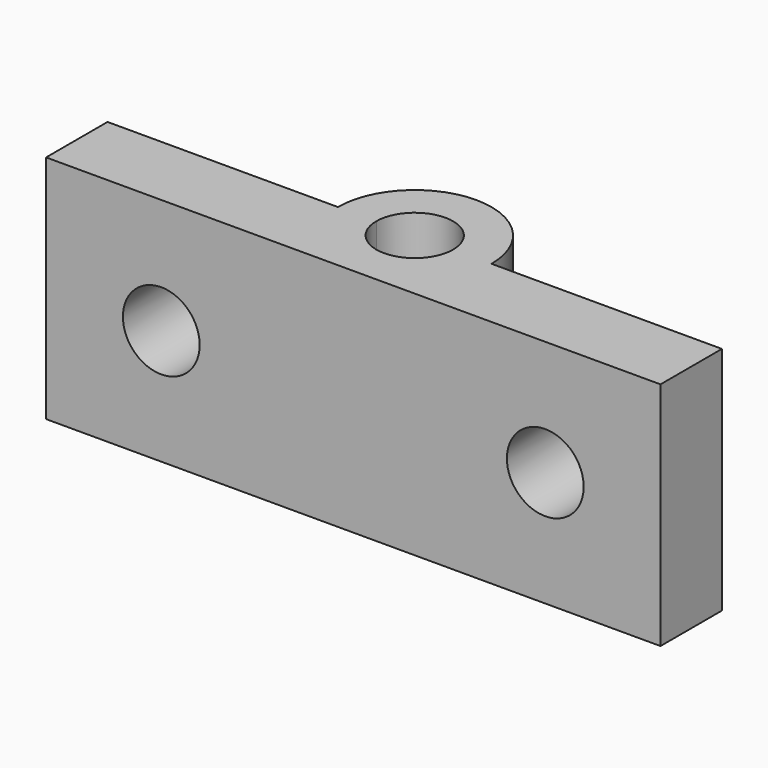
from build123d import *

# Parameters (mm, degrees)
F1_DEPTH = 9.525
F3_D     = 3.175
F5_D     = 3.175


# Not quite as in the source:
# - ends of sketch curves that miss each other by under 0.0002 mm in the source are joined
# - a length typed as a fraction of an inch, garbled in the dataset ("3 / 203.2 mm" for 3/8 in), is restored


with BuildPart() as f1:
    # F0 (on Top) → F1 (new body)
    with BuildSketch(Plane.XY):
        with BuildLine():
            ThreePointArc((7.6885502785, 1.9437116954), (5.4434862483, 1.0137757257), (4.5135502785, -1.2312883046))
            Line((4.5135502785, -1.2312883046), (6.1010502795, -1.2312883046))
            ThreePointArc((6.1010502795, -1.2312883046), (7.6885771705, 0.3561579113), (9.2760502785, -1.2313420884))
            Line((9.2760502785, -1.2313420884), (10.8635502785, -1.2312883046))
            ThreePointArc((10.8635502785, -1.2312883046), (9.9336143088, 1.0137757257), (7.6885502785, 1.9437116954))
        make_face()
        with BuildLine():
            Line((-5.0114497215, -1.2312883046), (-5.0114497215, -4.4062883046))
            Line((-5.0114497215, -4.4062883046), (20.3885502785, -4.4062883046))
            Line((20.3885502785, -4.4062883046), (20.3885502785, -1.2312883046))
            Line((20.3885502785, -1.2312883046), (10.8635502785, -1.2312883046))
            Line((10.8635502785, -1.2312883046), (9.2760502785, -1.2312883046))
            ThreePointArc((9.2760502785, -1.2312883046), (7.6885233866, -2.8188420882), (6.1010502795, -1.2312883046))
            Line((6.1010502795, -1.2312883046), (4.5135502785, -1.2312883046))
            Line((4.5135502785, -1.2312883046), (-5.0114497215, -1.2312883046))
        make_face()
    extrude(amount=F1_DEPTH)

    # F3 (through all)
    with Locations(Plane(origin=(0, -1.2312883046, 0), x_dir=(-1, 0, 0), z_dir=(0, 1, 0))):
        with Locations((-15.6260502785, 4.7625)):
            Hole(F3_D / 2)

    # F5 (through all)
    with Locations(Plane(origin=(0, -1.2312883046, 0), x_dir=(-1, 0, 0), z_dir=(0, 1, 0))):
        with Locations((0.2489497215, 4.7625)):
            Hole(F5_D / 2)


solid = f1.part
